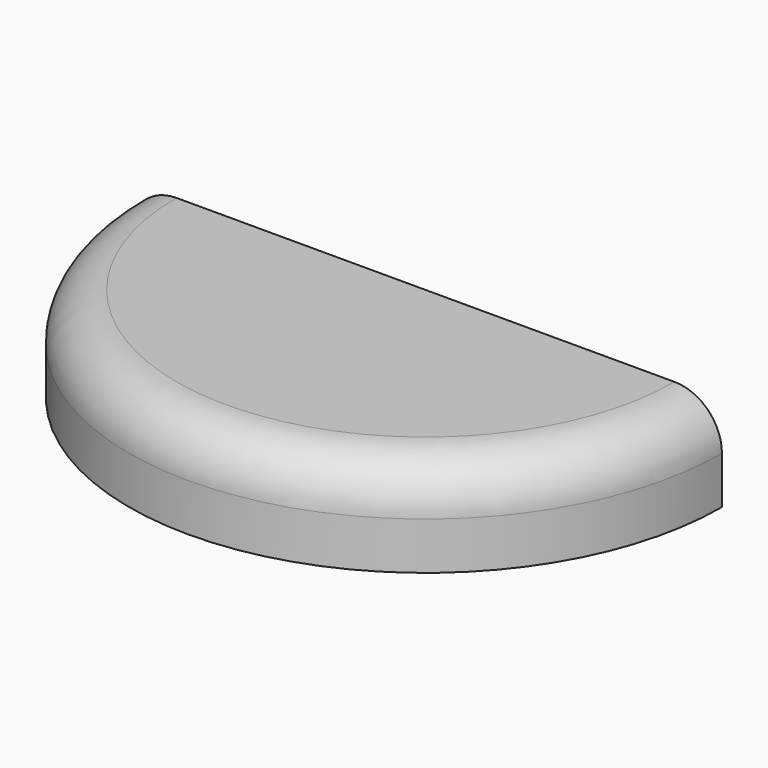
from build123d import *

# Parameters (mm, degrees)
F1_DEPTH = 2.54
F5_R     = 2.54


# Not quite as in the source:
# - the program builds the solid bodies; features that only make, move or delete a surface that nothing else refers to are left out


with BuildPart() as f1:
    # F0 (on Top) → F1 (new body, symmetric)
    with BuildSketch(Plane.XY):
        with BuildLine():
            ThreePointArc((-15.875, 0), (0, -15.875), (15.875, 0))
            Line((15.875, 0), (-15.875, 0))
        make_face()
    extrude(amount=F1_DEPTH, both=True)

    # F5
    f5_edges = [f1.edges().sort_by_distance(p)[0] for p in [
        (0, -15.875, 2.54),
    ]]
    fillet(f5_edges, radius=F5_R)


solid = f1.part
